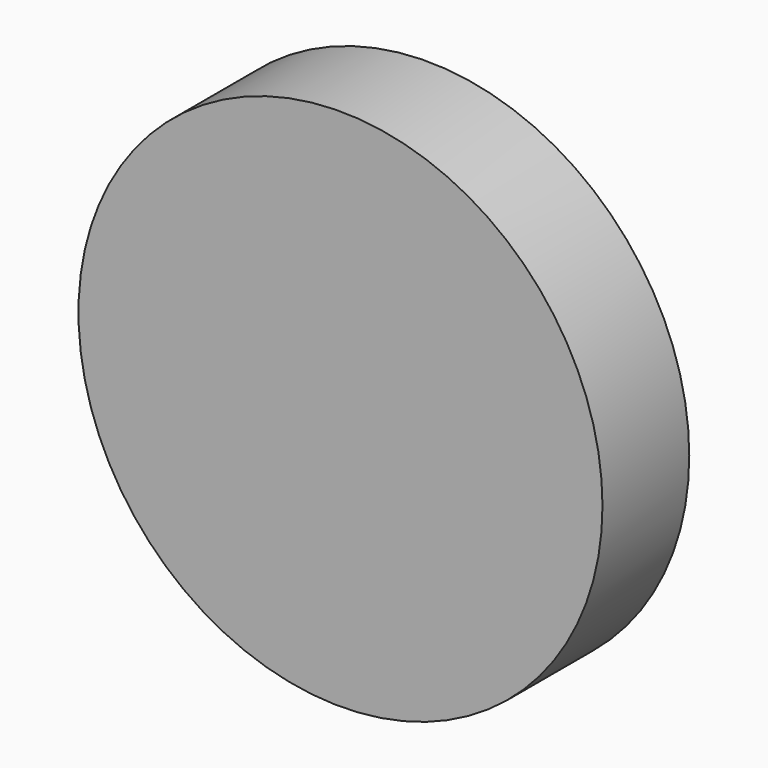
from build123d import *

# Parameters (mm, degrees)
F0_R     = 61.349245048
F2_DEPTH = 25.4
F1_R     = 61.349245048
F4_DEPTH = 25.4


# Not quite as in the source:
# - the program builds the solid bodies; features that only make, move or delete a surface that nothing else refers to are left out


with BuildPart() as f2:
    # F0 (on Front) → F2 (new body)
    with BuildSketch(Plane.XZ):
        Circle(F0_R)
    extrude(amount=F2_DEPTH)

    # F1 (on face) → F4 (join)
    with BuildSketch(Plane.XZ):
        Circle(F1_R)
    extrude(amount=F4_DEPTH)


solid = f2.part
